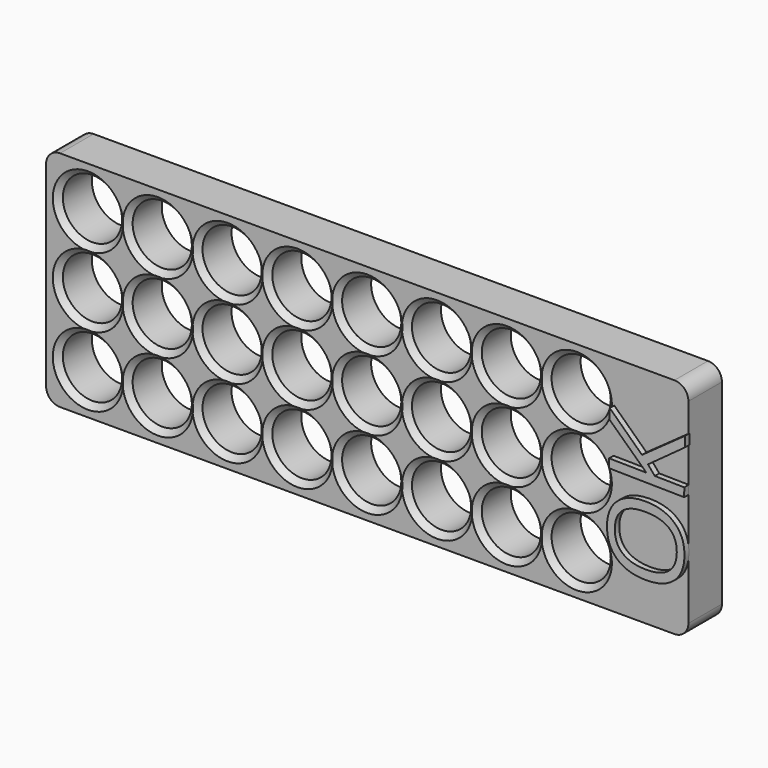
from build123d import *

# Parameters (mm, degrees)
F0_W         = 230
F0_H         = 80
F0_R         = 10.6
F1_DEPTH     = 15
F2_R         = 5
F4_TEXT_SIZE = 37.7219708818
F5_DEPTH     = 2


# Not quite as in the source:
# - a fillet or chamfer that OpenCascade refuses, or shapes differently, is made with other operations: its cross-section is extruded or revolved along the edge and cut away or added
# - a feature names something its author has since deleted; it is built from what else it names
# - Text() gives the source's letters only with a copy of the font that has no kerning and outlines rounded to 1/6400 em; it was checked with that copy


with BuildPart() as f1:
    # F0 (on Front) → F1 (new body)
    with BuildSketch(Plane.XZ):
        with Locations((10.2640186101, 115.6777501106)):
            Rectangle(F0_W, F0_H)
        with Locations((-89.7359813899, 90.6777501106)):
            Circle(F0_R, mode=Mode.SUBTRACT)
        with Locations((-64.7359813899, 90.6777501106)):
            Circle(F0_R, mode=Mode.SUBTRACT)
        with Locations((-39.7359813899, 90.6777501106)):
            Circle(F0_R, mode=Mode.SUBTRACT)
        with Locations((-14.7359813899, 90.6777501106)):
            Circle(F0_R, mode=Mode.SUBTRACT)
        with Locations((10.2640186101, 90.6777501106)):
            Circle(F0_R, mode=Mode.SUBTRACT)
        with Locations((-89.7359813899, 115.6777501106)):
            Circle(F0_R, mode=Mode.SUBTRACT)
        with Locations((-64.7359813899, 115.6777501106)):
            Circle(F0_R, mode=Mode.SUBTRACT)
        with Locations((-39.7359813899, 115.6777501106)):
            Circle(F0_R, mode=Mode.SUBTRACT)
        with Locations((-14.7359813899, 115.6777501106)):
            Circle(F0_R, mode=Mode.SUBTRACT)
        with Locations((10.2640186101, 115.6777501106)):
            Circle(F0_R, mode=Mode.SUBTRACT)
        with Locations((35.2640186101, 90.6777501106)):
            Circle(F0_R, mode=Mode.SUBTRACT)
        with Locations((60.2640186101, 90.6777501106)):
            Circle(F0_R, mode=Mode.SUBTRACT)
        with Locations((85.2640186101, 90.6777501106)):
            Circle(F0_R, mode=Mode.SUBTRACT)
        with Locations((35.2640186101, 115.6777501106)):
            Circle(F0_R, mode=Mode.SUBTRACT)
        with Locations((60.2640186101, 115.6777501106)):
            Circle(F0_R, mode=Mode.SUBTRACT)
        with Locations((85.2640186101, 115.6777501106)):
            Circle(F0_R, mode=Mode.SUBTRACT)
        with Locations((-89.7359813899, 140.6777501106)):
            Circle(F0_R, mode=Mode.SUBTRACT)
        with Locations((-64.7359813899, 140.6777501106)):
            Circle(F0_R, mode=Mode.SUBTRACT)
        with Locations((-39.7359813899, 140.6777501106)):
            Circle(F0_R, mode=Mode.SUBTRACT)
        with Locations((-14.7359813899, 140.6777501106)):
            Circle(F0_R, mode=Mode.SUBTRACT)
        with Locations((10.2640186101, 140.6777501106)):
            Circle(F0_R, mode=Mode.SUBTRACT)
        with Locations((35.2640186101, 140.6777501106)):
            Circle(F0_R, mode=Mode.SUBTRACT)
        with Locations((60.2640186101, 140.6777501106)):
            Circle(F0_R, mode=Mode.SUBTRACT)
        with Locations((85.2640186101, 140.6777501106)):
            Circle(F0_R, mode=Mode.SUBTRACT)
    extrude(amount=F1_DEPTH)

    # F2
    f2_edges = [f1.edges().sort_by_distance(p)[0] for p in [
        (125.264019, -7.5, 75.67775),
        (125.264019, -7.5, 155.67775),
        (-104.735981, -7.5, 155.67775),
        (-104.735981, -7.5, 75.67775),
    ]]
    fillet(f2_edges, radius=F2_R)

    # F3: chamfer of 2 on 24 edges, made by hand

    # F3_s1 → F3_t2 (revolve, cut)
    with BuildSketch(Plane.XY.offset(90.6777501106)):
        Polygon((-77.1359813899, -15), (-79.1359813899, -13), (-79.1359813899, -15), align=None)
    revolve(axis=Axis((-89.7359813899, -15, 90.6777501106), (0, -1, 0)), mode=Mode.SUBTRACT)

    # F3_s3 → F3_t4 (revolve, cut)
    with BuildSketch(Plane.XY.offset(115.6777501106)):
        Polygon((-77.1359813899, -15), (-79.1359813899, -13), (-79.1359813899, -15), align=None)
    revolve(axis=Axis((-89.7359813899, -15, 115.6777501106), (0, -1, 0)), mode=Mode.SUBTRACT)

    # F3_s5 → F3_t6 (revolve, cut)
    with BuildSketch(Plane.XY.offset(140.6777501106)):
        Polygon((-77.1359813899, -15), (-79.1359813899, -13), (-79.1359813899, -15), align=None)
    revolve(axis=Axis((-89.7359813899, -15, 140.6777501106), (0, -1, 0)), mode=Mode.SUBTRACT)

    # F3_s7 → F3_t8 (revolve, cut)
    with BuildSketch(Plane.XY.offset(140.6777501106)):
        Polygon((-52.1359813899, -15), (-54.1359813899, -13), (-54.1359813899, -15), align=None)
    revolve(axis=Axis((-64.7359813899, -15, 140.6777501106), (0, -1, 0)), mode=Mode.SUBTRACT)

    # F3_s9 → F3_t10 (revolve, cut)
    with BuildSketch(Plane.XY.offset(115.6777501106)):
        Polygon((-52.1359813899, -15), (-54.1359813899, -13), (-54.1359813899, -15), align=None)
    revolve(axis=Axis((-64.7359813899, -15, 115.6777501106), (0, -1, 0)), mode=Mode.SUBTRACT)

    # F3_s11 → F3_t12 (revolve, cut)
    with BuildSketch(Plane.XY.offset(90.6777501106)):
        Polygon((-52.1359813899, -15), (-54.1359813899, -13), (-54.1359813899, -15), align=None)
    revolve(axis=Axis((-64.7359813899, -15, 90.6777501106), (0, -1, 0)), mode=Mode.SUBTRACT)

    # F3_s13 → F3_t14 (revolve, cut)
    with BuildSketch(Plane.XY.offset(90.6777501106)):
        Polygon((-27.1359813899, -15), (-29.1359813899, -13), (-29.1359813899, -15), align=None)
    revolve(axis=Axis((-39.7359813899, -15, 90.6777501106), (0, -1, 0)), mode=Mode.SUBTRACT)

    # F3_s15 → F3_t16 (revolve, cut)
    with BuildSketch(Plane.XY.offset(115.6777501106)):
        Polygon((-27.1359813899, -15), (-29.1359813899, -13), (-29.1359813899, -15), align=None)
    revolve(axis=Axis((-39.7359813899, -15, 115.6777501106), (0, -1, 0)), mode=Mode.SUBTRACT)

    # F3_s17 → F3_t18 (revolve, cut)
    with BuildSketch(Plane.XY.offset(140.6777501106)):
        Polygon((-27.1359813899, -15), (-29.1359813899, -13), (-29.1359813899, -15), align=None)
    revolve(axis=Axis((-39.7359813899, -15, 140.6777501106), (0, -1, 0)), mode=Mode.SUBTRACT)

    # F3_s19 → F3_t20 (revolve, cut)
    with BuildSketch(Plane.XY.offset(140.6777501106)):
        Polygon((-2.1359813899, -15), (-4.1359813899, -13), (-4.1359813899, -15), align=None)
    revolve(axis=Axis((-14.7359813899, -15, 140.6777501106), (0, -1, 0)), mode=Mode.SUBTRACT)

    # F3_s21 → F3_t22 (revolve, cut)
    with BuildSketch(Plane.XY.offset(115.6777501106)):
        Polygon((-2.1359813899, -15), (-4.1359813899, -13), (-4.1359813899, -15), align=None)
    revolve(axis=Axis((-14.7359813899, -15, 115.6777501106), (0, -1, 0)), mode=Mode.SUBTRACT)

    # F3_s23 → F3_t24 (revolve, cut)
    with BuildSketch(Plane.XY.offset(90.6777501106)):
        Polygon((-2.1359813899, -15), (-4.1359813899, -13), (-4.1359813899, -15), align=None)
    revolve(axis=Axis((-14.7359813899, -15, 90.6777501106), (0, -1, 0)), mode=Mode.SUBTRACT)

    # F3_s25 → F3_t26 (revolve, cut)
    with BuildSketch(Plane.XY.offset(90.6777501106)):
        Polygon((22.8640186101, -15), (20.8640186101, -13), (20.8640186101, -15), align=None)
    revolve(axis=Axis((10.2640186101, -15, 90.6777501106), (0, -1, 0)), mode=Mode.SUBTRACT)

    # F3_s27 → F3_t28 (revolve, cut)
    with BuildSketch(Plane.XY.offset(115.6777501106)):
        Polygon((22.8640186101, -15), (20.8640186101, -13), (20.8640186101, -15), align=None)
    revolve(axis=Axis((10.2640186101, -15, 115.6777501106), (0, -1, 0)), mode=Mode.SUBTRACT)

    # F3_s29 → F3_t30 (revolve, cut)
    with BuildSketch(Plane.XY.offset(140.6777501106)):
        Polygon((22.8640186101, -15), (20.8640186101, -13), (20.8640186101, -15), align=None)
    revolve(axis=Axis((10.2640186101, -15, 140.6777501106), (0, -1, 0)), mode=Mode.SUBTRACT)

    # F3_s31 → F3_t32 (revolve, cut)
    with BuildSketch(Plane.XY.offset(140.6777501106)):
        Polygon((47.8640186101, -15), (45.8640186101, -13), (45.8640186101, -15), align=None)
    revolve(axis=Axis((35.2640186101, -15, 140.6777501106), (0, -1, 0)), mode=Mode.SUBTRACT)

    # F3_s33 → F3_t34 (revolve, cut)
    with BuildSketch(Plane.XY.offset(115.6777501106)):
        Polygon((47.8640186101, -15), (45.8640186101, -13), (45.8640186101, -15), align=None)
    revolve(axis=Axis((35.2640186101, -15, 115.6777501106), (0, -1, 0)), mode=Mode.SUBTRACT)

    # F3_s35 → F3_t36 (revolve, cut)
    with BuildSketch(Plane.XY.offset(140.6777501106)):
        Polygon((72.8640186101, -15), (70.8640186101, -13), (70.8640186101, -15), align=None)
    revolve(axis=Axis((60.2640186101, -15, 140.6777501106), (0, -1, 0)), mode=Mode.SUBTRACT)

    # F3_s37 → F3_t38 (revolve, cut)
    with BuildSketch(Plane.XY.offset(115.6777501106)):
        Polygon((72.8640186101, -15), (70.8640186101, -13), (70.8640186101, -15), align=None)
    revolve(axis=Axis((60.2640186101, -15, 115.6777501106), (0, -1, 0)), mode=Mode.SUBTRACT)

    # F3_s39 → F3_t40 (revolve, cut)
    with BuildSketch(Plane.XY.offset(140.6777501106)):
        Polygon((97.8640186101, -15), (95.8640186101, -13), (95.8640186101, -15), align=None)
    revolve(axis=Axis((85.2640186101, -15, 140.6777501106), (0, -1, 0)), mode=Mode.SUBTRACT)

    # F3_s41 → F3_t42 (revolve, cut)
    with BuildSketch(Plane.XY.offset(115.6777501106)):
        Polygon((97.8640186101, -15), (95.8640186101, -13), (95.8640186101, -15), align=None)
    revolve(axis=Axis((85.2640186101, -15, 115.6777501106), (0, -1, 0)), mode=Mode.SUBTRACT)

    # F3_s43 → F3_t44 (revolve, cut)
    with BuildSketch(Plane.XY.offset(90.6777501106)):
        Polygon((47.8640186101, -15), (45.8640186101, -13), (45.8640186101, -15), align=None)
    revolve(axis=Axis((35.2640186101, -15, 90.6777501106), (0, -1, 0)), mode=Mode.SUBTRACT)

    # F3_s45 → F3_t46 (revolve, cut)
    with BuildSketch(Plane.XY.offset(90.6777501106)):
        Polygon((72.8640186101, -15), (70.8640186101, -13), (70.8640186101, -15), align=None)
    revolve(axis=Axis((60.2640186101, -15, 90.6777501106), (0, -1, 0)), mode=Mode.SUBTRACT)

    # F3_s47 → F3_t48 (revolve, cut)
    with BuildSketch(Plane.XY.offset(90.6777501106)):
        Polygon((97.8640186101, -15), (95.8640186101, -13), (95.8640186101, -15), align=None)
    revolve(axis=Axis((85.2640186101, -15, 90.6777501106), (0, -1, 0)), mode=Mode.SUBTRACT)

    # F4 (on face) → F5 (join)
    with BuildSketch(Plane.XZ.offset(15)):
        with Locations(Location((124.8489320112, 88.1939451973), (0, 0, 89.1347303512))):
            Text('OK', F4_TEXT_SIZE, font='Open Sans', text_align=(TextAlign.LEFT, TextAlign.BOTTOM))
    extrude(amount=F5_DEPTH)


solid = f1.part
